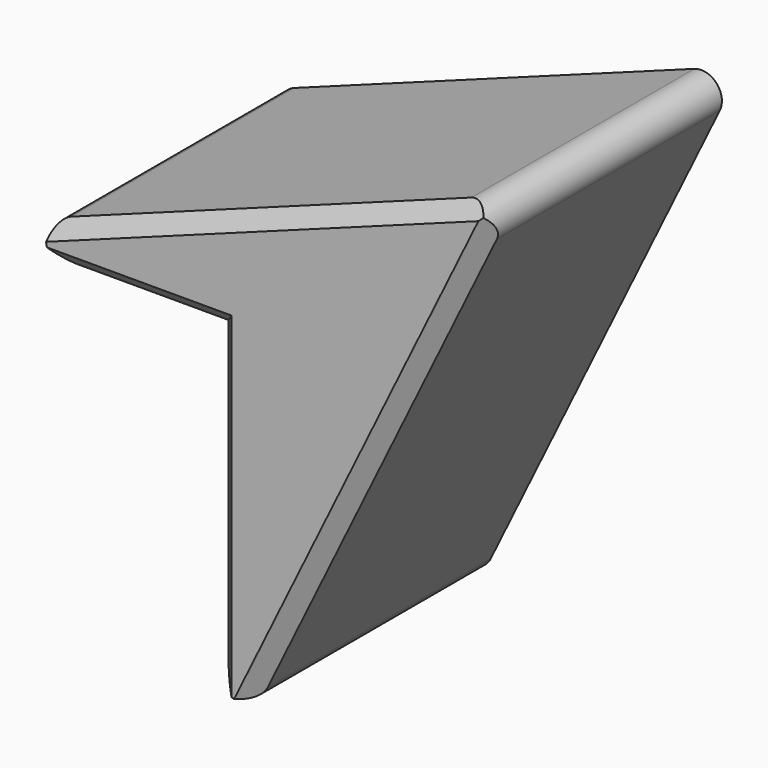
from build123d import *

# Parameters (mm, degrees)
F1_DEPTH    = 25.4
F2_SIZE     = 1.27
F3_T1_DEPTH = 62.588590634
F3_T3_DEPTH = 46.2433618017
F3_T5_DEPTH = 74.1232333831


# Not quite as in the source:
# - a fillet or chamfer that OpenCascade refuses, or shapes differently, is made with other operations: its cross-section is extruded or revolved along the edge and cut away or added


with BuildPart() as f1:
    # F0 (on Front) → F1 (new body)
    with BuildSketch(Plane.XZ):
        Polygon((0, 51.5181273222), (-48.1757372618, 33.8250361383), (-25.1621361822, 33.8250361383), (-25.1621361822, 0), align=None)
    extrude(amount=F1_DEPTH)

    # F2
    f2_edges = [f1.edges().sort_by_distance(p)[0] for p in [
        (-25.162136, -25.4, 16.912518),
        (-12.581068, -25.4, 25.759064),
        (-36.668937, -25.4, 33.825036),
        (-24.087869, -25.4, 42.671582),
    ]]
    chamfer(f2_edges, length=F2_SIZE)

    # F3: fillet of radius 1.778 on 3 edges, made by hand

    # F3_s2 → F3_t1 (cut)
    with BuildSketch(Plane.XZ.offset(-19.229295317)):
        with BuildLine():
            ThreePointArc((-21.78650907, 6.911415871), (-23.7845753127, 5.9593981498), (-25.1621361822, 7.6917181268))
            Line((-25.1621361822, 7.6917181268), (-25.1621361822, 0))
            Line((-25.1621361822, 0), (-21.78650907, 6.911415871))
        make_face()
    extrude(amount=F3_T1_DEPTH, mode=Mode.SUBTRACT)

    # F3_s4 → F3_t3 (cut)
    with BuildSketch(Plane.XZ.offset(-11.0566809008)):
        with BuildLine():
            ThreePointArc((-4.1515436611, 49.9934253721), (-2.2186732944, 49.5156925609), (-1.9409568164, 47.5441221078))
            Line((-1.9409568164, 47.5441221078), (0, 51.5181273222))
            Line((0, 51.5181273222), (-4.1515436611, 49.9934253721))
        make_face()
    extrude(amount=F3_T3_DEPTH, mode=Mode.SUBTRACT)

    # F3_s6 → F3_t5 (cut)
    with BuildSketch(Plane.XZ.offset(-24.9966166916)):
        with BuildLine():
            ThreePointArc((-38.7900503177, 37.2720371468), (-39.9276287585, 35.2917483238), (-38.1770905851, 33.8250361383))
            Line((-38.1770905851, 33.8250361383), (-48.1757372618, 33.8250361383))
            Line((-48.1757372618, 33.8250361383), (-38.7900503177, 37.2720371468))
        make_face()
    extrude(amount=F3_T5_DEPTH, mode=Mode.SUBTRACT)


solid = f1.part
